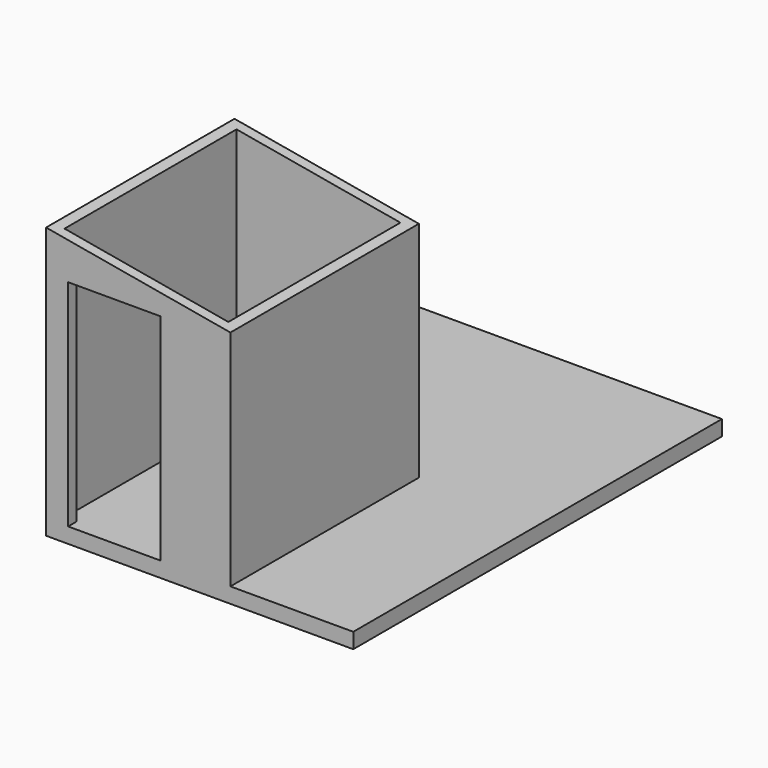
from build123d import *

# Parameters (mm, degrees)
F0_W      = 3000
F0_H      = 4500
F1_DEPTH  = 150
F2_W      = 1800
F2_H      = 2300
F2_W_2    = 1600
F2_H_2    = 2100
F4_DEPTH  = 2500
F6_DEPTH  = 2300
F7_W      = 900
F7_H      = 2100
F8_DEPTH  = 800
F9_W      = 300
F9_H      = 500
F10_DEPTH = 100


# Not quite as in the source:
# - a feature of the source that left no trace in its solid (it failed there, or was rolled back) is left out


with BuildPart() as f1:
    # F0 (on Top) → F1 (new body)
    with BuildSketch(Plane.XY):
        Rectangle(F0_W, F0_H)
    extrude(amount=F1_DEPTH)

    # F2 (on face) → F4 (join)
    with BuildSketch(Plane.XY.offset(150)):
        with Locations((-600, -1100)):
            Rectangle(F2_W, F2_H)
        with Locations((-600, -1100)):
            Rectangle(F2_W_2, F2_H_2, mode=Mode.SUBTRACT)
    extrude(amount=F4_DEPTH)

    # F5 (on face) → F6 (cut, through all)
    with BuildSketch(Plane.XZ.offset(2250)):
        Polygon((300, 2650), (-1500, 2650), (300, 2332.6114347248), align=None)
    extrude(amount=-F6_DEPTH, mode=Mode.SUBTRACT)

    # F7 (on face) → F8 (cut)
    with BuildSketch(Plane.XZ.offset(2250)):
        with Locations((-835, 1200)):
            Rectangle(F7_W, F7_H)
    extrude(amount=-F8_DEPTH, mode=Mode.SUBTRACT)

    # F9 (on face) → F10 (cut, through all)
    with BuildSketch(Plane(origin=(0, 50, 0), x_dir=(-1, 0, 0), z_dir=(0, 1, 0))):
        with Locations((-50, 400)):
            Rectangle(F9_W, F9_H)
    extrude(amount=-F10_DEPTH, mode=Mode.SUBTRACT)


solid = f1.part
